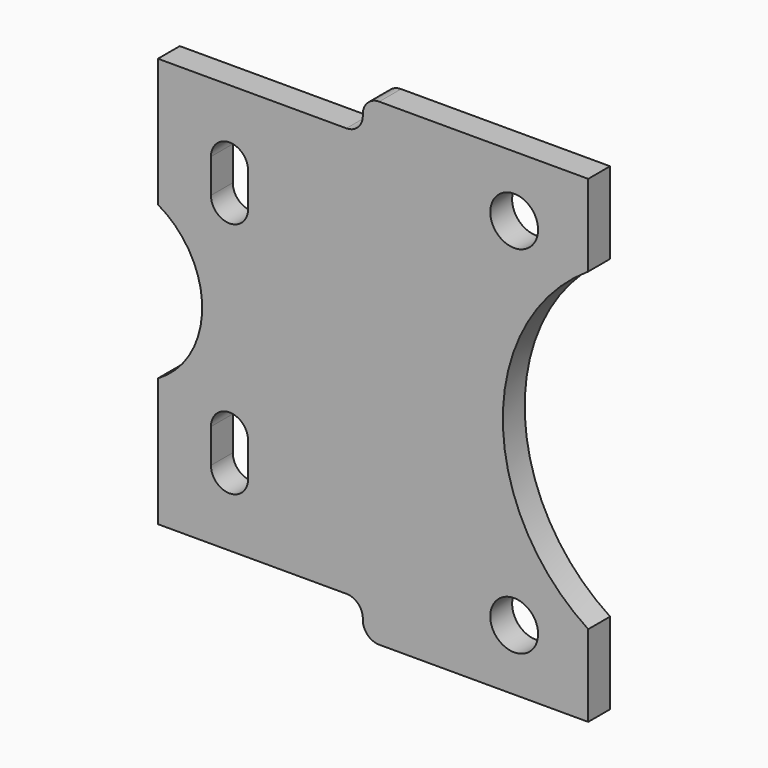
from build123d import *

# Parameters (mm, degrees)
F0_W     = 30.48
F0_H     = 2.54
F1_DEPTH = 44.45
F0_W_2   = 9.525
F3_DEPTH = 44.45
F4_R     = 2.2225
F5_DEPTH = 25.4
F2_W     = 19.05
F2_H     = 3.175
F6_DEPTH = 25.4
F7_R     = 1.524


# Not quite as in the source:
# - a feature names something its author has since deleted; it is built from what else it names


with BuildPart() as f1:
    # F0 (on Top) → F1 (new body)
    with BuildSketch(Plane.XY):
        with Locations((-15.24, 1.27)):
            Rectangle(F0_W, F0_H)
    extrude(amount=F1_DEPTH)

    # F0 (on Top) → F3 (join)
    with BuildSketch(Plane.XY):
        with Locations((4.7625, 1.27)):
            Rectangle(F0_W_2, F0_H)
    extrude(amount=F3_DEPTH)

    # F4 (on face) + F2 (on face) → F5 (cut)
    with BuildSketch(Plane.XZ):
        with Locations((2.6416, 38.7731)):
            Circle(F4_R)
        with Locations((2.6416, 5.6769)):
            Circle(F4_R)
        with BuildLine():
            Line((9.525, 7.588973174), (9.525, 36.861026826))
            ThreePointArc((9.525, 36.861026826), (1.5875, 22.225), (9.525, 7.588973174))
        make_face()
    with BuildSketch(Plane.XZ):
        with BuildLine():
            Line((-22.098, 9.5885), (-22.098, 12.7635))
            ThreePointArc((-22.098, 12.7635), (-23.8252, 14.4907), (-25.5524, 12.7635))
            Line((-25.5524, 12.7635), (-25.5524, 9.5885))
            ThreePointArc((-25.5524, 9.5885), (-23.8252, 7.8613), (-22.098, 9.5885))
        make_face()
        with BuildLine():
            Line((-22.098, 31.6865), (-22.098, 34.8615))
            ThreePointArc((-22.098, 34.8615), (-23.8252, 36.5887), (-25.5524, 34.8615))
            Line((-25.5524, 34.8615), (-25.5524, 31.6865))
            ThreePointArc((-25.5524, 31.6865), (-23.8252, 29.9593), (-22.098, 31.6865))
        make_face()
        with BuildLine():
            Line((-30.48, 29.337), (-30.48, 15.113))
            ThreePointArc((-30.48, 15.113), (-26.3652, 22.225), (-30.48, 29.337))
        make_face()
    extrude(amount=-F5_DEPTH, mode=Mode.SUBTRACT)

    # F2 (on face) → F6 (cut)
    with BuildSketch(Plane.XZ):
        with Locations((-20.955, 42.8625)):
            Rectangle(F2_W, F2_H)
        with Locations((-20.955, 1.5875)):
            Rectangle(F2_W, F2_H)
    extrude(amount=-F6_DEPTH, mode=Mode.SUBTRACT)

    # F7
    f7_edges = [f1.edges().sort_by_distance(p)[0] for p in [
        (-11.43, 1.27, 41.275),
        (-11.43, 1.27, 44.45),
        (-11.43, 1.27, 0),
        (-11.43, 1.27, 3.175),
    ]]
    fillet(f7_edges, radius=F7_R)


solid = f1.part
